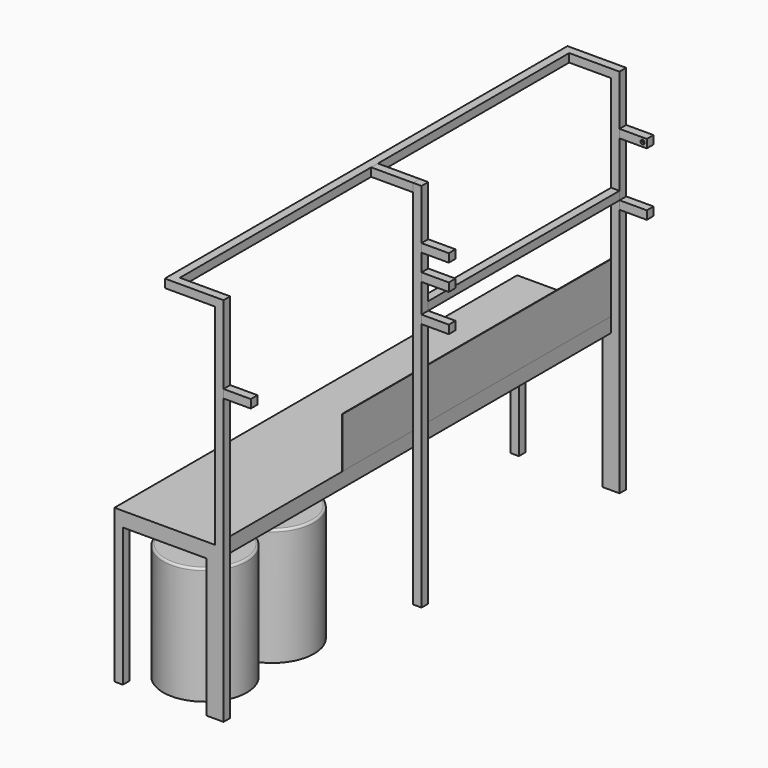
from build123d import *

# Parameters (mm, degrees)
F0_W      = 3048
F0_H      = 88.9
F1_DEPTH  = 609.6
F2_W      = 50.8
F2_H      = 50.8
F3_DEPTH  = 838.2
F5_DEPTH  = 711.2
F6_W      = 50.8
F6_H      = 50.8
F7_DEPTH  = 2247.9
F8_W      = 3048
F8_H      = 50.8
F9_DEPTH  = 304.8
F10_W     = 254
F10_H     = 2946.4
F11_DEPTH = 50.8
F12_W     = 3.175
F12_H     = 2032
F13_DEPTH = 304.8
F14_W     = 50.8
F14_H     = 50.8
F15_DEPTH = 2247.9
F16_T     = -25.4
F17_T     = -25.4
F18_R     = 12.69999
F19_R     = 12.69999
F20_W     = 50.8
F20_H     = 50.8
F21_DEPTH = 1447.8
F22_W     = 50.8
F22_H     = 50.8
F23_DEPTH = 165.1
F24_W     = 50.8
F24_H     = 50.8
F25_DEPTH = 254
F26_W     = 50.8
F26_H     = 50.8
F27_DEPTH = 165.1
F28_W     = 50.8
F28_H     = 50.8
F29_DEPTH = 165.1
F31_D     = 25.4
F31_DEPTH = 12.7
F31_TIP   = 7.6309298617
F33_D     = 25.4
F33_DEPTH = 12.7
F33_TIP   = 7.6309298617


# Not quite as in the source:
# - a fillet or chamfer is up to 0.001 mm smaller than in the source, because OpenCascade refuses the exact size


with BuildPart() as f1:
    # F0 (on Right) → F1 (new body)
    with BuildSketch(Plane.YZ):
        with Locations((183.6904625475, -73.3985408201)):
            Rectangle(F0_W, F0_H)
    extrude(amount=-F1_DEPTH)

    # F2 (on face) → F3 (join)
    with BuildSketch(Plane(origin=(0, 0, -117.8485408201), x_dir=(1, 0, 0), z_dir=(0, 0, -1))):
        with Locations((-584.2, 1314.9095374525)):
            Rectangle(F2_W, F2_H)
        with Locations((-25.4, 1314.9095374525)):
            Rectangle(F2_W, F2_H)
        with Locations((-25.4, -1682.2904625475)):
            Rectangle(F2_W, F2_H)
        with Locations((-584.2, -1682.2904625475)):
            Rectangle(F2_W, F2_H)
    extrude(amount=F3_DEPTH)

    # F6 (on face) → F7 (join)
    with BuildSketch(Plane(origin=(0, 0, -956.0485408201), x_dir=(1, 0, 0), z_dir=(0, 0, -1))):
        with Locations((25.4, 1314.9095374525)):
            Rectangle(F6_W, F6_H)
        with Locations((25.4, -1682.2904625475)):
            Rectangle(F6_W, F6_H)
    extrude(amount=-F7_DEPTH)

    # F8 (on face) → F9 (join)
    with BuildSketch(Plane(origin=(0, 0, 0), x_dir=(0, -1, 0), z_dir=(-1, 0, 0))):
        with Locations((-183.6904625475, 1266.4514591799)):
            Rectangle(F8_W, F8_H)
    extrude(amount=F9_DEPTH)

    # F10 (on face) → F11 (cut, through all)
    with BuildSketch(Plane.XY.offset(1291.8514591799)):
        with Locations((-127, 183.6904625475)):
            Rectangle(F10_W, F10_H)
    extrude(amount=-F11_DEPTH, mode=Mode.SUBTRACT)


with BuildPart() as f5:
    # F4 (on face) → F5 (new body)
    with BuildSketch(Plane(origin=(0, 0, -956.0485408201), x_dir=(1, 0, 0), z_dir=(0, 0, -1))):
        with BuildLine():
            ThreePointArc((-304.8, 781.5095374525), (-125.1948775786, 855.9044150311), (-50.8, 1035.5095374525))
            ThreePointArc((-50.8, 1035.5095374525), (-484.4051224214, 1215.1146598738), (-304.8, 781.5095374525))
        make_face()
    extrude(amount=-F5_DEPTH)

    # F17
    f17_openings = [f5.faces().sort_by_distance(p)[0] for p in [
        (-304.8, -1035.509537, -244.848541),
    ]]
    offset(amount=F17_T, openings=f17_openings)

    # F18 (radius 12.7 in the source; OpenCascade refuses exactly that, so slightly less here)
    f18_edges = [f5.edges().sort_by_distance(p)[0] for p in [
        (-304.8, -1289.509537, -244.848541),
        (-304.8, -1264.109537, -244.848541),
    ]]
    fillet(f18_edges, radius=F18_R)


with BuildPart() as f5b:
    # F4 (on face) → F5, piece 2 (new body)
    with BuildSketch(Plane(origin=(0, 0, -956.0485408201), x_dir=(1, 0, 0), z_dir=(0, 0, -1))):
        with BuildLine():
            ThreePointArc((-50.8, 527.5095374525), (-125.1948775786, 707.1146598738), (-304.8, 781.5095374525))
            ThreePointArc((-304.8, 781.5095374525), (-484.4051224214, 347.9044150311), (-50.8, 527.5095374525))
        make_face()
    extrude(amount=-F5_DEPTH)

    # F16
    f16_openings = [f5b.faces().sort_by_distance(p)[0] for p in [
        (-304.8, -527.509537, -244.848541),
    ]]
    offset(amount=F16_T, openings=f16_openings)

    # F19 (radius 12.7 in the source; OpenCascade refuses exactly that, so slightly less here)
    f19_edges = [f5b.edges().sort_by_distance(p)[0] for p in [
        (-558.8, -527.509537, -244.848541),
        (-533.4, -527.509537, -244.848541),
    ]]
    fillet(f19_edges, radius=F19_R)


with BuildPart() as f13:
    # F12 (on face) → F13 (new body)
    with BuildSketch(Plane.XY.offset(-28.9485408201)):
        with Locations((-1.5875, 640.8904625475)):
            Rectangle(F12_W, F12_H)
    extrude(amount=F13_DEPTH)


with BuildPart() as f15:
    # F14 (on face) → F15 (new body)
    with BuildSketch(Plane(origin=(0, 0, -956.0485408201), x_dir=(1, 0, 0), z_dir=(0, 0, -1))):
        with Locations((25.4, -183.6904625475)):
            Rectangle(F14_W, F14_H)
    extrude(amount=-F15_DEPTH)


with BuildPart() as f21:
    # F20 (on face) → F21 (new body, through all)
    with BuildSketch(Plane.XZ.offset(-1656.8904625475)):
        with Locations((25.4, 631.4514591799)):
            Rectangle(F20_W, F20_H)
    extrude(amount=F21_DEPTH)


with BuildPart() as f23:
    # F22 (on face) → F23 (new body)
    with BuildSketch(Plane.YZ.offset(50.8)):
        with Locations((183.6904625475, 805.7018689156)):
            Rectangle(F22_W, F22_H)
    extrude(amount=F23_DEPTH)


with BuildPart() as f23b:
    # F22 (on face) → F23, piece 2 (new body)
    with BuildSketch(Plane.YZ.offset(50.8)):
        with Locations((-1314.9095374525, 793.3480314255)):
            Rectangle(F22_W, F22_H)
    extrude(amount=F23_DEPTH)


with BuildPart() as f25:
    # F24 (on face) → F25 (new body, through all)
    with BuildSketch(Plane(origin=(0, 0, 0), x_dir=(0, -1, 0), z_dir=(-1, 0, 0))):
        with Locations((-183.6904625475, 1266.4514591799)):
            Rectangle(F24_W, F24_H)
    extrude(amount=F25_DEPTH)


with BuildPart() as f27:
    # F26 (on face) → F27 (new body)
    with BuildSketch(Plane.YZ.offset(50.8)):
        with Locations((183.6904625475, 580.6514591799)):
            Rectangle(F26_W, F26_H)
    extrude(amount=F27_DEPTH)


with BuildPart() as f27b:
    # F26 (on face) → F27, piece 2 (new body)
    with BuildSketch(Plane.YZ.offset(50.8)):
        with Locations((1682.7640108109, 580.6514591799)):
            Rectangle(F26_W, F26_H)
    extrude(amount=F27_DEPTH)


with BuildPart() as f29:
    # F28 (on face) → F29 (new body)
    with BuildSketch(Plane.YZ.offset(50.8)):
        with Locations((183.6904625475, 961.6514591799)):
            Rectangle(F28_W, F28_H)
    extrude(amount=F29_DEPTH)

    # F33
    with Locations(Plane(origin=(0, 209.0904625475, 0), x_dir=(-1, 0, 0), z_dir=(0, 1, 0))):
        with Locations((-190.5, 961.6514591799)):
            Hole(F33_D / 2, depth=F33_DEPTH)
            with Locations((0, 0, -(F33_DEPTH + F33_TIP / 2))):  # 118° drill point
                Cone(0, F33_D / 2, F33_TIP, mode=Mode.SUBTRACT)


with BuildPart() as f29b:
    # F28 (on face) → F29, piece 2 (new body)
    with BuildSketch(Plane.YZ.offset(50.8)):
        with Locations((1682.2904625475, 961.6514591799)):
            Rectangle(F28_W, F28_H)
    extrude(amount=F29_DEPTH)

    # F31
    with Locations(Plane.XZ.offset(-1656.8904625475)):
        with Locations((190.5, 961.6514591799)):
            Hole(F31_D / 2, depth=F31_DEPTH)
            with Locations((0, 0, -(F31_DEPTH + F31_TIP / 2))):  # 118° drill point
                Cone(0, F31_D / 2, F31_TIP, mode=Mode.SUBTRACT)


solid = Compound([f1.part, f5.part, f5b.part, f13.part, f15.part, f21.part, f23.part, f23b.part, f25.part, f27.part, f27b.part, f29.part, f29b.part])
